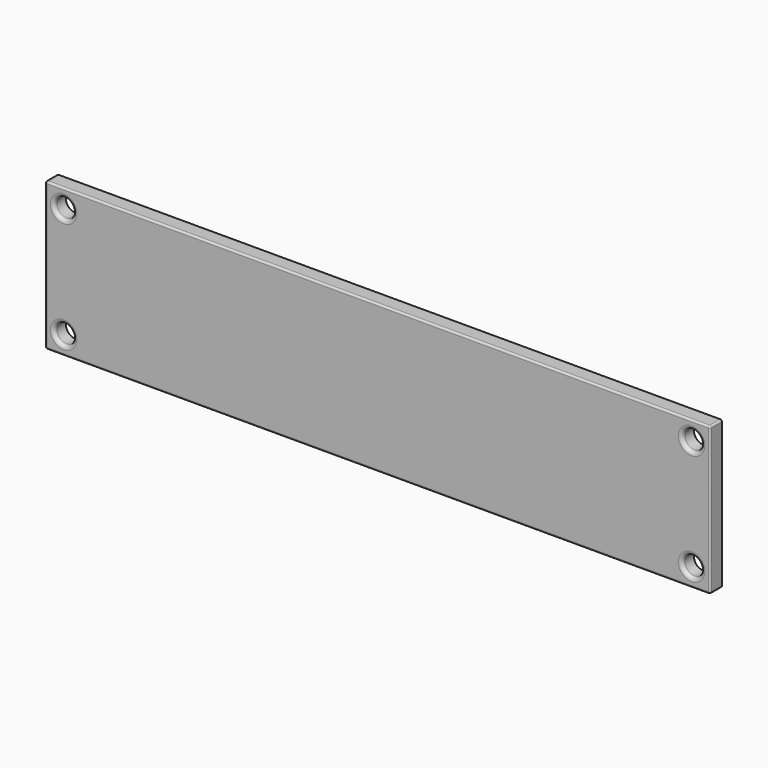
from build123d import *

# Parameters (mm, degrees)
F0_W     = 180
F0_H     = 40
F0_R     = 2.5751263091
F1_DEPTH = 4
F2_R     = 1
F3_R     = 0.5


# Not quite as in the source:
# - a feature names something its author has since deleted; it is built from what else it names


with BuildPart() as f1:
    # F0 (on Front) → F1 (new body)
    with BuildSketch(Plane.XZ):
        Rectangle(F0_W, F0_H)
        with Locations((-85, -15)):
            Circle(F0_R, mode=Mode.SUBTRACT)
        with Locations((85, -15)):
            Circle(F0_R, mode=Mode.SUBTRACT)
        with Locations((-85, 15)):
            Circle(F0_R, mode=Mode.SUBTRACT)
        with Locations((85, 15)):
            Circle(F0_R, mode=Mode.SUBTRACT)
    extrude(amount=F1_DEPTH)

    # F2
    f2_edges = [f1.edges().sort_by_distance(p)[0] for p in [
        (-87.575126, -4, 15),
        (-87.575126, -4, -15),
        (82.424874, -4, 15),
        (82.424874, -4, -15),
    ]]
    fillet(f2_edges, radius=F2_R)

    # F3
    f3_edges = [f1.edges().sort_by_distance(p)[0] for p in [
        (0, -4, 20),
        (-90, -4, 0),
        (0, -4, -20),
        (90, -4, 0),
        (-90, -2, 20),
        (-90, -2, -20),
        (90, -2, 20),
        (90, -2, -20),
    ]]
    fillet(f3_edges, radius=F3_R)


solid = f1.part
